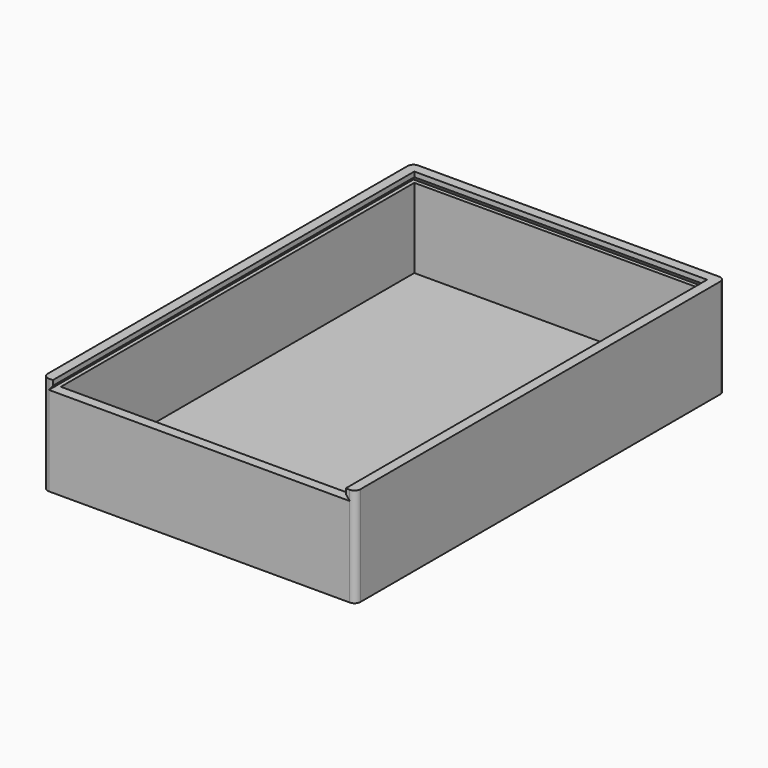
from build123d import *

# Parameters (mm, degrees)
F0_W     = 63
F0_H     = 18
F1_DEPTH = 93
F2_T     = -2
F4_DEPTH = 93
F6_DEPTH = 63
F7_R     = 1.19999


# Not quite as in the source:
# - a fillet or chamfer is up to 0.001 mm smaller than in the source, because OpenCascade refuses the exact size


with BuildPart() as f1:
    # F0 (on Front) → F1 (new body)
    with BuildSketch(Plane.XZ):
        with Locations((31.5, -9)):
            Rectangle(F0_W, F0_H)
    extrude(amount=-F1_DEPTH)

    # F2
    f2_openings = [f1.faces().sort_by_distance(p)[0] for p in [
        (31.5, 46.5, 0),
    ]]
    offset(amount=F2_T, openings=f2_openings)

    # F3 (on face) → F4 (join, through all)
    with BuildSketch(Plane.XZ):
        Polygon((0, 2), (0, 0), (1.2, 0), (2, 1), (2, 2), align=None)
        Polygon((61, 1), (61.8, 0), (63, 0), (63, 2), (61, 2), align=None)
    extrude(amount=-F4_DEPTH)

    # F5 (on face) → F6 (join, through all)
    with BuildSketch(Plane.YZ.offset(63)):
        Polygon((93, 0), (93, 2), (91, 2), (91, 1), (91.8, 0), align=None)
    extrude(amount=-F6_DEPTH)

    # F7 (radius 1.2 in the source; OpenCascade refuses exactly that, so slightly less here)
    f7_edges = [f1.edges().sort_by_distance(p)[0] for p in [
        (63, 0, -8),
        (63, 93, -8),
        (0, 0, -8),
        (0, 93, -8),
    ]]
    fillet(f7_edges, radius=F7_R)


solid = f1.part
